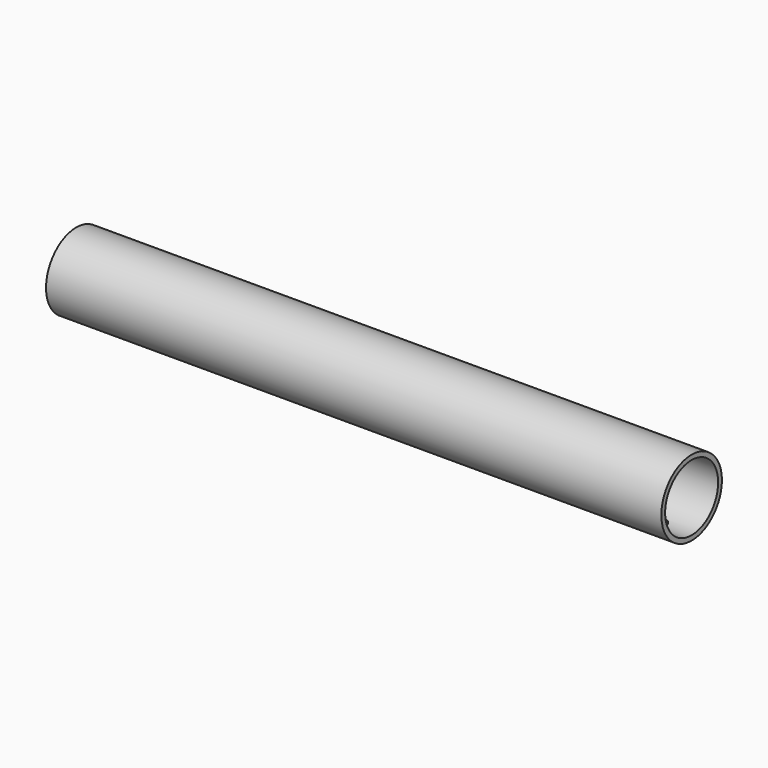
from build123d import *

# Parameters (mm, degrees)
F0_R     = 8
F0_R_2   = 7
F1_DEPTH = 65
F2_W     = 10
F2_H     = 10
F3_DEPTH = 25
F4_R     = 1
F5_R     = 1.6
F6_DEPTH = 25


# Not quite as in the source:
# - a pattern or mirror of a feature is missing from the dataset's text; its kind, count and spacing are read off the source's solid


with BuildPart() as f1:
    # F0 (on Right) → F1 (new body, symmetric)
    with BuildSketch(Plane.YZ):
        Circle(F0_R)
        Circle(F0_R_2, mode=Mode.SUBTRACT)
    extrude(amount=F1_DEPTH, both=True)

    # F2 (on Front) → F3 (cut)
    with BuildSketch(Plane.XZ):
        Rectangle(F2_W, F2_H)
    extrude(amount=-F3_DEPTH, mode=Mode.SUBTRACT)

    # F4
    f4_edges = [f1.edges().sort_by_distance(p)[0] for p in [
        (-5, 5.571989, -5),
        (5, 5.571989, -5),
        (5, 5.571989, 5),
        (-5, 5.571989, 5),
    ]]
    fillet(f4_edges, radius=F4_R)

    # F5 (on Top) → F6 (cut)
    with BuildSketch(Plane.XY):
        with Locations((-58, 0)):
            Circle(F5_R)
    f6 = extrude(amount=-F6_DEPTH, mode=Mode.SUBTRACT)

    # F6_copies: F6 across plane
    add(f6.mirror(Plane(origin=(-4e-06, 0, 0), x_dir=(0, 0, 1), z_dir=(1, 0, 0))), mode=Mode.SUBTRACT)


solid = f1.part
